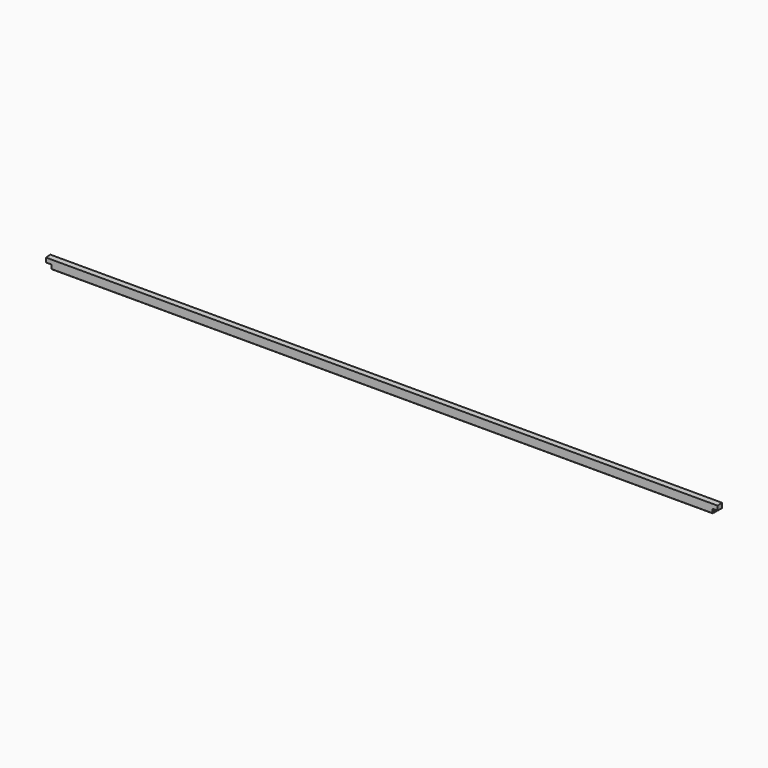
from build123d import *

# Parameters (mm, degrees)
F1_DEPTH      = 2550
F2_W          = 80
F2_H          = 66
F3_DEPTH      = 50
F6_DEPTH      = 2550.001
F6_DEPTH_BACK = 2550.001


with BuildPart() as f1:
    # F0 (on Right) → F1 (new body, symmetric)
    with BuildSketch(Plane.YZ):
        Polygon((20, -70), (20, 56), (17, 59), (12, 59), (12, 73), (4, 73), (4, 59), (-4, 59), (-4, 73), (-12, 73), (-12, 59), (-17, 59), (-20, 56), (-20, -70), (-17, -73), (-12, -73), (-12, -59), (-4, -59), (-4, -73), (4, -73), (4, -59), (12, -59), (12, -73), (17, -73), align=None)
    extrude(amount=F1_DEPTH, both=True)

    # F2 (on Front) → F3 (cut, symmetric)
    with BuildSketch(Plane.XZ):
        with Locations((-2550, 59)):
            Rectangle(F2_W, F2_H)
        with Locations((-2550, -73)):
            Rectangle(F2_W, F2_H)
        with Locations((2550, 59)):
            Rectangle(F2_W, F2_H)
        with Locations((2550, -73)):
            Rectangle(F2_W, F2_H)
    extrude(amount=F3_DEPTH, both=True, mode=Mode.SUBTRACT)

    # F5 (on Right) → F6 (cut, two sides)
    with BuildSketch(Plane.YZ) as f6_sk:
        Polygon((30, -2.3176279375), (30, 83), (-30, 83), (-30, -7.9364744125), align=None)
    extrude(amount=-F6_DEPTH, mode=Mode.SUBTRACT)
    extrude(f6_sk.sketch, amount=F6_DEPTH_BACK, mode=Mode.SUBTRACT)


solid = f1.part
